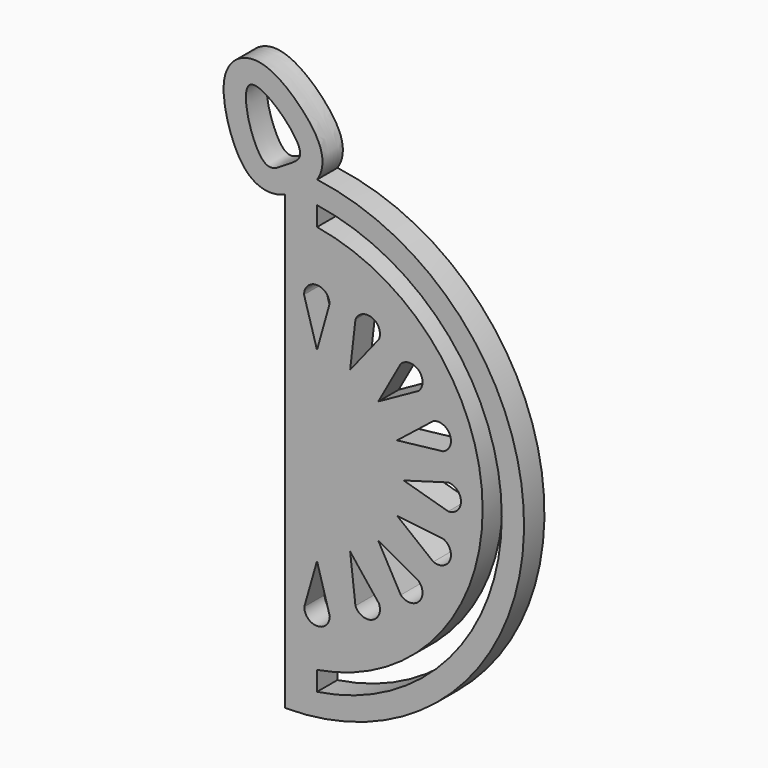
from build123d import *

# Parameters (mm, degrees)
F1_DEPTH = 1.016


# Not quite as in the source:
# - the dataset's text gives a spline's control points without its knots; the knots are read off the source's solid
# - a feature names something its author has since deleted; it is built from what else it names


with BuildPart() as f1:
    # F0 (on Front) → F1 (new body)
    with BuildSketch(Plane.XZ):
        with BuildLine():
            Line((0.8720639816, 7.9696412083), (0.8720639816, -10.0599602319))
            ThreePointArc((0.8720639816, -10.0599602319), (10.3756166469, -1.17379647), (2.1468595371, 8.9043470145))
            add(Edge.make_bspline(
                [(2.1468595371, 8.9043470145), (2.1375619429, 8.8904589251), (2.0865405168, 8.8173483885), (1.9460704833, 8.6552218776), (1.7420457163, 8.4951357663), (1.5810849761, 8.3938358775), (1.4761600351, 8.3297187682), (1.4351295268, 8.3042443679), (1.4146787791, 8.2911748332)],
                knots=[0.8870857839, 0.8870857839, 0.8870857839, 0.8870857839, 0.890625, 0.90625, 0.9375, 0.96875, 0.984375, 1, 1, 1, 1], degree=3))
            add(Edge.make_bspline(
                [(1.4146787791, 8.2911748332), (1.3942280315, 8.2781052984), (1.3534555492, 8.2513015595), (1.2501088251, 8.1821845952), (1.1037829859, 8.0867078461), (0.9512588202, 8.0042801492), (0.8720639816, 7.9696412083)],
                knots=[0, 0, 0, 0, 0.015625, 0.03125, 0.0625, 0.0871949279, 0.0871949279, 0.0871949279, 0.0871949279], degree=3))
        make_face()
        with BuildLine():
            Line((2.1420639816, -4.4827677338), (2.6500639816, -6.2599216028))
            ThreePointArc((2.6500639816, -6.2599216028), (2.1420639816, -6.7679216028), (1.6340639816, -6.2599216028))
            Line((1.6340639816, -6.2599216028), (2.1420639816, -4.4827677338))
        make_face(mode=Mode.SUBTRACT)
        with BuildLine():
            Line((3.4634338013, -3.7250291716), (4.6131757466, -5.1732837967))
            ThreePointArc((4.6131757466, -5.1732837967), (4.3382481277, -5.8370177829), (3.6745141416, -5.562090164))
            Line((3.6745141416, -5.562090164), (3.4634338013, -3.7250291716))
        make_face(mode=Mode.SUBTRACT)
        with BuildLine():
            Line((4.5836370443, -2.9765332945), (6.2000831461, -3.8745589066))
            ThreePointArc((6.2000831461, -3.8745589066), (6.2000831461, -4.5929793963), (5.4816626564, -4.5929793963))
            Line((5.4816626564, -4.5929793963), (4.5836370443, -2.9765332945))
        make_face(mode=Mode.SUBTRACT)
        with BuildLine():
            Line((5.3321329213, -1.8563300516), (7.1691939138, -2.0674103918))
            ThreePointArc((7.1691939138, -2.0674103918), (7.4441215326, -2.731144378), (6.7803875465, -3.0060719968))
            Line((6.7803875465, -3.0060719968), (5.3321329213, -1.8563300516))
        make_face(mode=Mode.SUBTRACT)
        with BuildLine():
            ThreePointArc((2.1420639816, 8.0071470023), (9.5080639816, -0.5349602319), (2.1420639816, -9.077067466))
            Line((2.1420639816, -9.077067466), (2.1420639816, -8.3058659706))
            ThreePointArc((2.1420639816, -8.3058659706), (8.7460639816, -0.5349602319), (2.1420639816, 7.2359455069))
            Line((2.1420639816, 7.2359455069), (2.1420639816, 8.0071470023))
        make_face(mode=Mode.SUBTRACT)
        with BuildLine():
            Line((5.5949697203, -0.5349602319), (7.3729697203, -0.0269602319))
            ThreePointArc((7.3729697203, -0.0269602319), (7.8809697203, -0.5349602319), (7.3729697203, -1.0429602319))
            Line((7.3729697203, -1.0429602319), (5.5949697203, -0.5349602319))
        make_face(mode=Mode.SUBTRACT)
        with BuildLine():
            Line((5.3321329213, 0.7864095879), (6.7803875465, 1.9361515331))
            ThreePointArc((6.7803875465, 1.9361515331), (7.4441215326, 1.6612239143), (7.1691939138, 0.9974899281))
            Line((7.1691939138, 0.9974899281), (5.3321329213, 0.7864095879))
        make_face(mode=Mode.SUBTRACT)
        with BuildLine():
            Line((2.1420639816, 2.9179455069), (1.6247334216, 4.6932531117))
            ThreePointArc((1.6247334216, 4.6932531117), (2.1327404272, 5.2012601173), (2.6407474328, 4.6932531117))
            Line((2.6407474328, 4.6932531117), (2.1420639816, 2.9179455069))
        make_face(mode=Mode.SUBTRACT)
        with BuildLine():
            Line((3.4634338013, 2.6551087078), (3.6745141416, 4.4921697003))
            ThreePointArc((3.6745141416, 4.4921697003), (4.3382481277, 4.7670973191), (4.6131757466, 4.103363333))
            Line((4.6131757466, 4.103363333), (3.4634338013, 2.6551087078))
        make_face(mode=Mode.SUBTRACT)
        with BuildLine():
            Line((4.5836370443, 1.9066128308), (5.4816626564, 3.5230589326))
            ThreePointArc((5.4816626564, 3.5230589326), (6.200083146, 3.5230589326), (6.2000831461, 2.8046384429))
            Line((6.2000831461, 2.8046384429), (4.5836370443, 1.9066128308))
        make_face(mode=Mode.SUBTRACT)
        with BuildLine():
            add(Edge.make_bspline(
                [(2.1468595371, 8.9043470145), (2.1375619429, 8.8904589251), (2.0865405168, 8.8173483885), (1.9460704833, 8.6552218776), (1.7420457163, 8.4951357663), (1.5810849761, 8.3938358775), (1.4761600351, 8.3297187682), (1.4351295268, 8.3042443679), (1.4146787791, 8.2911748332)],
                knots=[0.8870857839, 0.8870857839, 0.8870857839, 0.8870857839, 0.890625, 0.90625, 0.9375, 0.96875, 0.984375, 1, 1, 1, 1], degree=3))
            ThreePointArc((2.1468595371, 8.9043470145), (1.5109002197, 8.9685924334), (0.8720639816, 8.9900397681))
            Line((0.8720639816, 8.9900397681), (0.8720639816, 7.9696412083))
            add(Edge.make_bspline(
                [(1.4146787791, 8.2911748332), (1.3942280315, 8.2781052984), (1.3534555492, 8.2513015595), (1.2501088251, 8.1821845952), (1.1037829859, 8.0867078461), (0.9512588202, 8.0042801492), (0.8720639816, 7.9696412083)],
                knots=[0, 0, 0, 0, 0.015625, 0.03125, 0.0625, 0.0871949279, 0.0871949279, 0.0871949279, 0.0871949279], degree=3))
        make_face()
        with BuildLine():
            ThreePointArc((0.8720639816, 8.9900397681), (1.5109002197, 8.9685924334), (2.1468595371, 8.9043470145))
            add(Edge.make_bspline(
                [(0.8720639816, 7.9696412083), (0.8510423418, 7.960446577), (0.7249813726, 7.9081278301), (0.5036077396, 7.8428386533), (0.1763517707, 7.8396617002), (-0.0823939536, 7.8915061916), (-0.3251654939, 7.9972515694), (-0.5341027476, 8.1434171752), (-0.697739214, 8.3044391135), (-0.8691513012, 8.5179837512), (-1.0380674288, 8.7949781885), (-1.2052049627, 9.1500571037), (-1.3450151386, 9.5258501154), (-1.4577963792, 9.9145311538), (-1.5401925336, 10.3079754275), (-1.5788115991, 10.635693281), (-1.5852425405, 10.9015252067), (-1.5741785001, 11.1062228204), (-1.5405553236, 11.3219253664), (-1.4704609064, 11.5567984789), (-1.33596904, 11.8170093575), (-1.1321876014, 12.0375341588), (-0.908583488, 12.1756170372), (-0.6774819455, 12.2669258051), (-0.4050529119, 12.3032860953), (-0.1378640903, 12.2767253775), (0.0853156063, 12.2174366098), (0.2811335851, 12.13963355), (0.5205476797, 12.0186949927), (0.7961357942, 11.8411620626), (1.1088534794, 11.5949546296), (1.4042104843, 11.3229328113), (1.6775187355, 11.0325659825), (1.9220461866, 10.7287576582), (2.0970325204, 10.463495283), (2.216248269, 10.2308639089), (2.3198947054, 9.9728588144), (2.3801931706, 9.6400082363), (2.3303267053, 9.292286109), (2.248064936, 9.0708356121), (2.1786091427, 8.9517723325), (2.1468595371, 8.9043470145)],
                knots=[0.0871949279, 0.0871949279, 0.0871949279, 0.0871949279, 0.09375, 0.125, 0.140625, 0.15625, 0.171875, 0.1875, 0.203125, 0.21875, 0.25, 0.28125, 0.3125, 0.34375, 0.375, 0.40625, 0.421875, 0.4375, 0.453125, 0.46875, 0.484375, 0.5, 0.5078125, 0.515625, 0.53125, 0.546875, 0.5625, 0.578125, 0.59375, 0.625, 0.65625, 0.6875, 0.71875, 0.75, 0.78125, 0.796875, 0.8125, 0.84375, 0.859375, 0.875, 0.8870857839, 0.8870857839, 0.8870857839, 0.8870857839], degree=3))
            Line((0.8720639816, 7.9696412083), (0.8720639816, 8.9900397681))
        make_face()
        with BuildLine():
            add(Edge.make_bspline(
                [(0.9359423365, 9.0402629925), (0.6263213587, 8.8423866229), (-0.161252366, 8.1539099286), (-1.4674404396, 12.930843348), (2.0880429138, 9.6009320246), (1.23446335, 9.2310454608), (0.9359423365, 9.0402629925)],
                knots=[0, 0, 0, 0, 0.1884203182, 0.5040626137, 0.8183345821, 1, 1, 1, 1], degree=3))
        make_face(mode=Mode.SUBTRACT)
    extrude(amount=F1_DEPTH)


solid = f1.part
